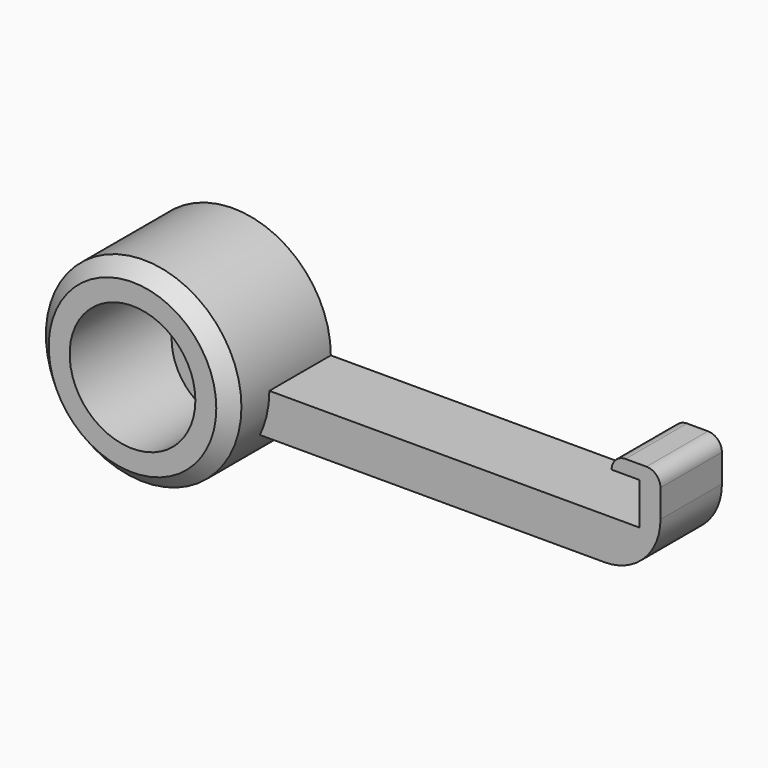
from build123d import *

# Parameters (mm, degrees)
F1_DEPTH = 5.5
F2_R     = 0.99999
F3_R     = 4
F4_R     = 7
F4_R_2   = 4.5
F5_DEPTH = 9
F6_SIZE  = 1


# Not quite as in the source:
# - a fillet or chamfer is up to 0.001 mm smaller than in the source, because OpenCascade refuses the exact size


with BuildPart() as f1:
    # F0 (on Front) → F1 (new body)
    with BuildSketch(Plane.XZ):
        Polygon((0, 4), (0, 0), (1.5, 0), (1.5, 3), (3.5, 3), (3.5, 4), align=None)
        Polygon((1.5, 0), (0, 0), (0, -3), (35, -3), (35, 0), (33.5, 0), (17.5, 0), align=None)
        Polygon((33.5, 3), (33.5, 0), (35, 0), (35, 4), (31.5, 4), (31.5, 3), align=None)
    extrude(amount=F1_DEPTH)

    # F2 (radius 1 in the source; OpenCascade refuses exactly that, so slightly less here)
    f2_edges = [f1.edges().sort_by_distance(p)[0] for p in [
        (31.5, -2.75, 4),
        (3.5, -2.75, 4),
        (35, -2.75, 4),
        (0, -2.75, 4),
    ]]
    fillet(f2_edges, radius=F2_R)

    # F3
    f3_edges = [f1.edges().sort_by_distance(p)[0] for p in [
        (0, -2.75, -3),
        (35, -2.75, -3),
    ]]
    fillet(f3_edges, radius=F3_R)


with BuildPart() as f5:
    # F4 (on Front) → F5 (new body)
    with BuildSketch(Plane.XZ):
        Circle(F4_R)
        Circle(F4_R_2, mode=Mode.SUBTRACT)
    extrude(amount=F5_DEPTH)

    # F6
    f6_edges = [f5.edges().sort_by_distance(p)[0] for p in [
        (-7, -9, 0),
    ]]
    chamfer(f6_edges, length=F6_SIZE)


solid = Compound([f1.part, f5.part])
